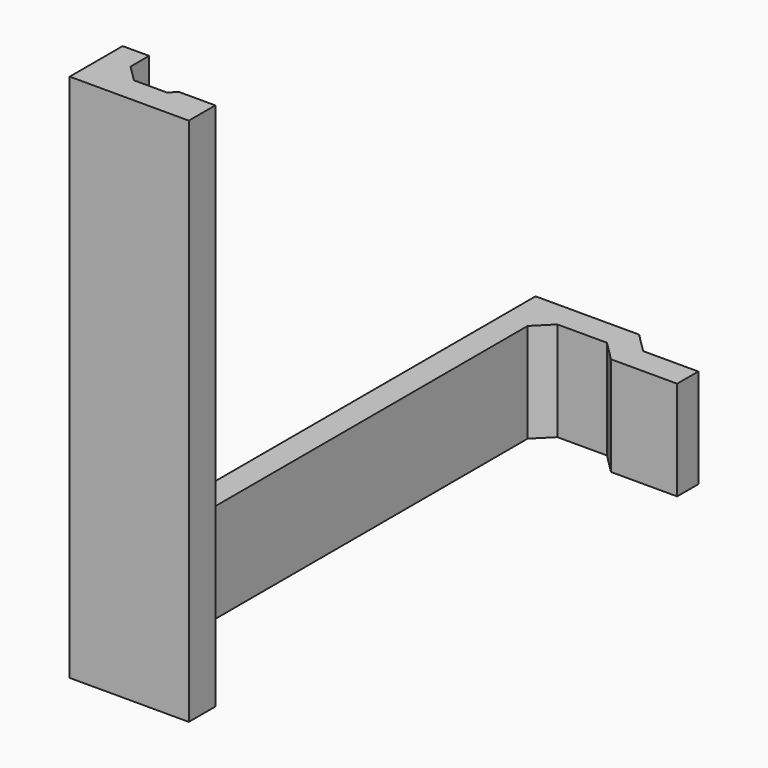
from build123d import *

# Parameters (mm, degrees)
F1_DEPTH    = 15
F3_DEPTH    = 65
F4_T1_DEPTH = 15
F4_T3_DEPTH = 80
F4_T8_DEPTH = 80


# Not quite as in the source:
# - a fillet or chamfer that OpenCascade refuses, or shapes differently, is made with other operations: its cross-section is extruded or revolved along the edge and cut away or added
# - a feature names something its author has since deleted; it is built from what else it names


with BuildPart() as f1:
    # F0 (on Top) → F1 (new body)
    with BuildSketch(Plane.XY):
        Polygon((0, 88), (0, 0), (18, 0), (18, 5), (14, 5), (14, 4), (4, 4), (4, 84), (14, 84), (17, 81), (27, 81), (27, 85), (18.6568542495, 85), (15.6568542495, 88), align=None)
    extrude(amount=F1_DEPTH)

    # F2 (on face) → F3 (join)
    with BuildSketch(Plane.XY.offset(15)):
        Polygon((4, 10), (0, 10), (0, 0), (18, 0), (18, 5), (14, 5), (14, 4), (4, 4), align=None)
    extrude(amount=F3_DEPTH)

    # F4: chamfer of 2.5 on 3 edges, made by hand

    # F4_s2 → F4_t1 (join)
    with BuildSketch(Plane.XY):
        Polygon((6.5, 84), (4, 81.5), (4, 84), align=None)
    extrude(amount=F4_T1_DEPTH)

    # F4_s4 → F4_t3 (join)
    with BuildSketch(Plane.XY):
        Polygon((4, 6.5), (6.5, 4), (4, 4), align=None)
    extrude(amount=F4_T3_DEPTH)


with BuildPart() as f4_tool6:
    # F4_s7 → F4_t8 (new body)
    with BuildSketch(Plane.XY):
        Polygon((11.5, 4), (14, 6.5), (14, 4), align=None)
    extrude(amount=F4_T8_DEPTH)

    split(bisect_by=Plane.XZ.offset(-5), keep=Keep.TOP)


with BuildPart() as f1_1:
    add(f1.part)

    # F4_t5: union F4_tool6
    add(f4_tool6.part)


solid = f1_1.part
